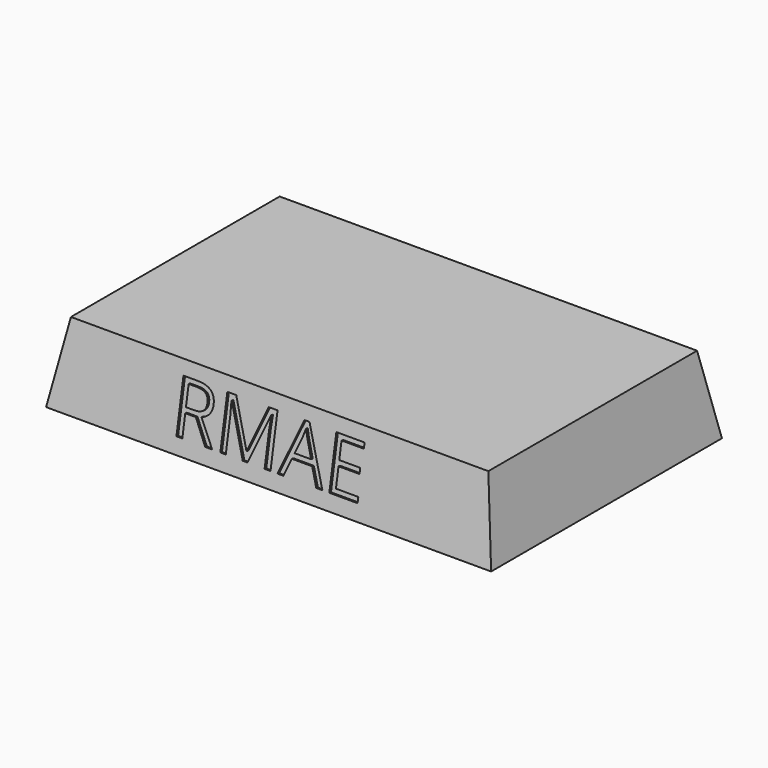
from build123d import *

# Parameters (mm, degrees)
F0_W         = 400
F0_H         = 250
F1_DEPTH     = 75
F1_TAPER     = -10
F2_TEXT_SIZE = 68.0174471603
F3_DEPTH     = 2


# Not quite as in the source:
# - Text() gives the source's letters only with a copy of the font that has no kerning and outlines rounded to 1/6400 em; it was checked with that copy


with BuildPart() as f1:
    # F0 (on Top) → F1 (new body)
    with BuildSketch(Plane.XY):
        Rectangle(F0_W, F0_H)
    extrude(amount=-F1_DEPTH, taper=F1_TAPER)

    # F2 (on face) → F3 (cut)
    with BuildSketch(Plane(origin=(0, -121.2307887991, 21.3762589579), x_dir=(1, 0, 0), z_dir=(0, -0.984807753, 0.1736481777))):
        with Locations((-97.0033556223, -83.3290219307)):
            Text('RMAE', F2_TEXT_SIZE, font='Open Sans', text_align=(TextAlign.LEFT, TextAlign.BOTTOM))
    extrude(amount=-F3_DEPTH, mode=Mode.SUBTRACT)


solid = f1.part
